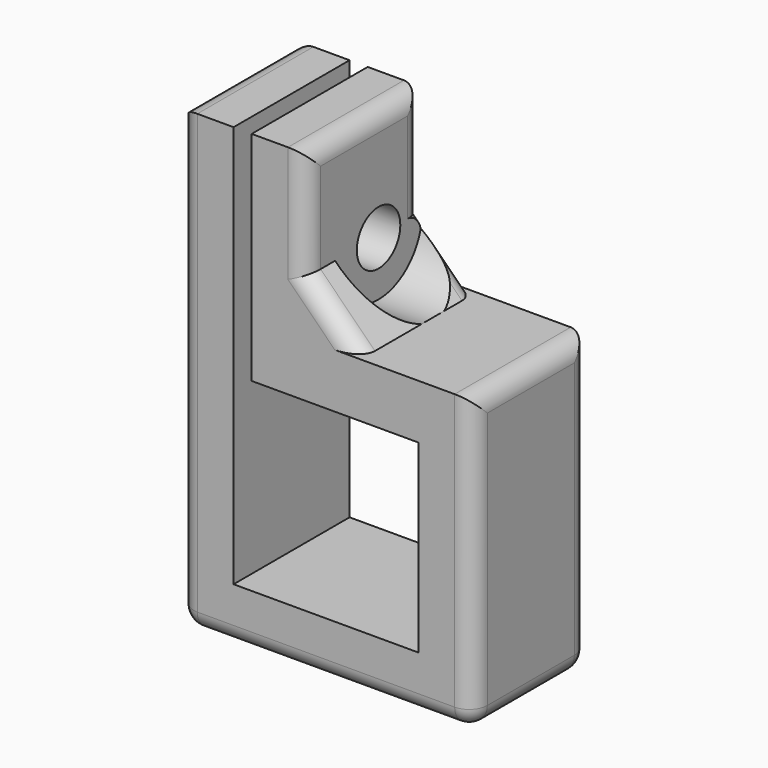
from build123d import *

# Parameters (mm, degrees)
F1_DEPTH    = 8
F2_R        = 1.5
F3_DEPTH    = 7.001
F4_T4_DEPTH = 8
F4_S5_R     = 1.5
F4_T6_DEPTH = 6
F5_R        = 1
F6_R        = 1
F7_R        = 3
F8_DEPTH    = 3


# Not quite as in the source:
# - a fillet or chamfer that OpenCascade refuses, or shapes differently, is made with other operations: its cross-section is extruded or revolved along the edge and cut away or added


with BuildPart() as f1:
    # F0 (on Front) → F1 (new body)
    with BuildSketch(Plane.XZ):
        Polygon((5.1, 5.1), (5.1, -5.1), (-5.1, -5.1), (-5.1, 5.1), (-5.1, 8.1), (-5.1, 17.1), (-8.1, 17.1), (-8.1, 8.1), (-8.1, -8.1), (8.1, -8.1), (8.1, 8.1), (-1.1, 8.1), (-1.1, 17.1), (-4.1, 17.1), (-4.1, 8.1), (-4.1, 5.1), align=None)
    extrude(amount=F1_DEPTH)

    # F2 (on face) → F3 (cut, through all)
    with BuildSketch(Plane.YZ.offset(-1.1)):
        with Locations((-3, 11)):
            Circle(F2_R)
    extrude(amount=-F3_DEPTH, mode=Mode.SUBTRACT)

    # F4: chamfer of 3 on 1 edges, made by hand


with BuildPart() as f4_tool2:
    # F4_s3 → F4_t4 (new body)
    with BuildSketch(Plane.XZ):
        Polygon((1.9, 8.1), (-1.1, 11.1), (-1.1, 8.1), align=None)
    extrude(amount=F4_T4_DEPTH)

    # F4_s5 → F4_t6 (cut, symmetric)
    with BuildSketch(Plane.YZ.offset(0.4)):
        with Locations((-3, 11)):
            Circle(F4_S5_R)
    extrude(amount=F4_T6_DEPTH, both=True, mode=Mode.SUBTRACT)


with BuildPart() as f1_1:
    add(f1.part)

    # F4_t1: union F4_tool2
    add(f4_tool2.part)

    # F5
    f5_edges = [f1_1.edges().sort_by_distance(p)[0] for p in [
        (8.1, -4, -8.1),
        (8.1, -4, 8.1),
        (8.1, 0, 0),
        (8.1, -8, 0),
        (-8.1, -4, -8.1),
        (0, 0, -8.1),
        (0, -8, -8.1),
        (-8.1, -4, 17.1),
        (-8.1, 0, 4.5),
        (-8.1, -8, 4.5),
        (-1.1, -4, 17.1),
        (-1.1, 0, 14.1),
        (-1.1, -8, 14.1),
    ]]
    fillet(f5_edges, radius=F5_R)

    # F6
    f6_edges = [f1_1.edges().sort_by_distance(p)[0] for p in [
        (0.4, 0, 9.6),
        (0.4, -8, 9.6),
    ]]
    fillet(f6_edges, radius=F6_R)

    # F7 (on face) → F8 (cut)
    with BuildSketch(Plane.YZ.offset(-1.1)):
        with Locations((-3, 11)):
            Circle(F7_R)
    extrude(amount=F8_DEPTH, mode=Mode.SUBTRACT)


solid = f1_1.part
